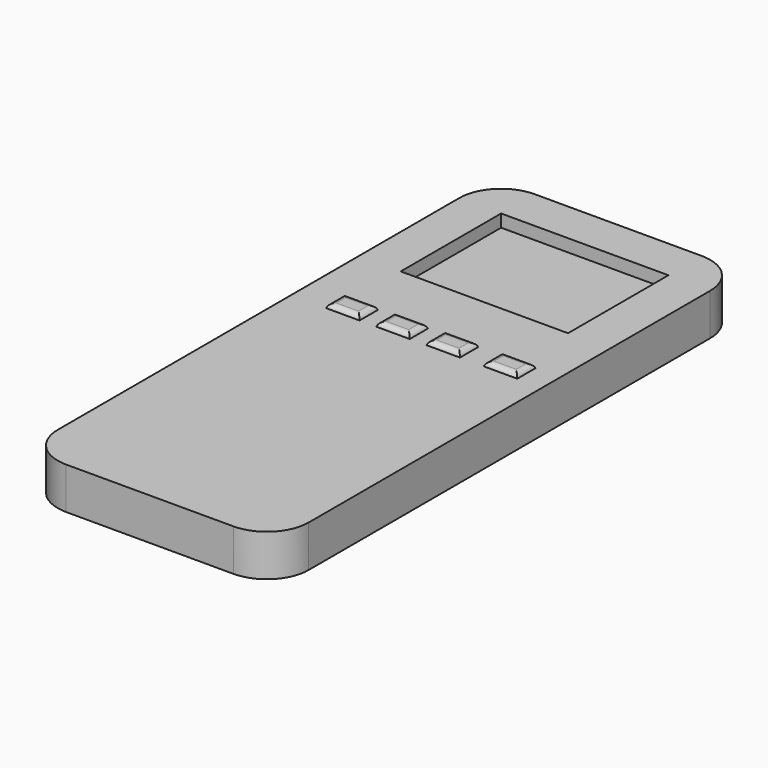
from build123d import *

# Parameters (mm, degrees)
F0_W        = 50.8
F0_H        = 38.1
F1_DEPTH    = 12.7
F2_DEPTH    = 8.89
F3_W        = 10.16
F3_H        = 6.9189891219
F3_H_2      = 6.9088
F4_DEPTH    = 1.27
F5_T1_DEPTH = 18.6794189943
F5_T3_DEPTH = 15.4384081162
F6_T1_DEPTH = 15.4384081162
F6_T3_DEPTH = 18.6794189943
F6_T5_DEPTH = 18.6794189943
F6_T7_DEPTH = 18.6794189943
F6_T9_DEPTH = 15.4282189943


# Not quite as in the source:
# - a fillet or chamfer that OpenCascade refuses, or shapes differently, is made with other operations: its cross-section is extruded or revolved along the edge and cut away or added


with BuildPart() as f1:
    # F0 (on Top) → F1 (new body)
    with BuildSketch(Plane.XY):
        with BuildLine():
            Line((26.8096346408, 46.6933250427), (-49.3903653592, 46.6933250427))
            Line((-49.3903653592, 46.6933250427), (-49.3903653592, -52.5104318142))
            ThreePointArc((-49.3903653592, -52.5104318142), (-45.6706214803, -61.4906879353), (-36.6903653592, -65.2104318142))
            Line((-36.6903653592, -65.2104318142), (14.1096346408, -65.2104318142))
            ThreePointArc((14.1096346408, -65.2104318142), (23.0898907619, -61.4906879353), (26.8096346408, -52.5104318142))
            Line((26.8096346408, -52.5104318142), (26.8096346408, 46.6933250427))
        make_face()
        with BuildLine():
            Line((14.1096346408, 112.5895681858), (-36.6903653592, 112.5895681858))
            ThreePointArc((-36.6903653592, 112.5895681858), (-45.6706214803, 108.8698243069), (-49.3903653592, 99.8895681858))
            Line((-49.3903653592, 99.8895681858), (-49.3903653592, 46.6933250427))
            Line((-49.3903653592, 46.6933250427), (26.8096346408, 46.6933250427))
            Line((26.8096346408, 46.6933250427), (26.8096346408, 99.8895681858))
            ThreePointArc((26.8096346408, 99.8895681858), (23.0898907619, 108.8698243069), (14.1096346408, 112.5895681858))
        make_face()
        with Locations((-11.2903653592, 80.8395681858)):
            Rectangle(F0_W, F0_H, mode=Mode.SUBTRACT)
    extrude(amount=F1_DEPTH)

    # F0 (on Top) → F2 (join)
    with BuildSketch(Plane.XY):
        with Locations((-11.2903653592, 80.8395681858)):
            Rectangle(F0_W, F0_H)
    extrude(amount=F2_DEPTH)

    # F3 (on face) → F4 (join)
    with BuildSketch(Plane.XY.offset(12.7)):
        with Locations((-33.6411841828, 39.4687093794)):
            Rectangle(F3_W, F3_H)
        with Locations((-18.4011841828, 39.4687093794)):
            Rectangle(F3_W, F3_H)
        with Locations((-3.1611841828, 39.4738039404)):
            Rectangle(F3_W, F3_H_2)
        with Locations((14.2273069042, 39.4738039404)):
            Rectangle(F3_W, F3_H_2)
    extrude(amount=F4_DEPTH)

    # F5: fillet of radius 1.778 on 4 edges, made by hand

    # F5_s2 → F5_t1 (cut)
    with BuildSketch(Plane.YZ.offset(-42.9808936799)):
        with BuildLine():
            ThreePointArc((42.9282039404, 12.7), (42.2868783752, 13.6175714644), (41.2243201415, 13.97))
            Line((41.2243201415, 13.97), (42.9282039404, 13.97))
            Line((42.9282039404, 13.97), (42.9282039404, 12.7))
        make_face()
        with BuildLine():
            ThreePointArc((36.0092148185, 12.7), (36.6505403836, 13.6175714644), (37.7130986173, 13.97))
            Line((37.7130986173, 13.97), (36.0092148185, 13.97))
            Line((36.0092148185, 13.97), (36.0092148185, 12.7))
        make_face()
    extrude(amount=F5_T1_DEPTH, mode=Mode.SUBTRACT)

    # F5_s4 → F5_t3 (cut)
    with BuildSketch(Plane.XZ.offset(-47.1879134375)):
        with BuildLine():
            ThreePointArc((-38.7211841828, 12.7), (-38.0798586176, 13.6175714644), (-37.0173003839, 13.97))
            Line((-37.0173003839, 13.97), (-38.7211841828, 13.97))
            Line((-38.7211841828, 13.97), (-38.7211841828, 12.7))
        make_face()
        with BuildLine():
            ThreePointArc((-28.5611841828, 12.7), (-29.2025097479, 13.6175714644), (-30.2650679816, 13.97))
            Line((-30.2650679816, 13.97), (-28.5611841828, 13.97))
            Line((-28.5611841828, 13.97), (-28.5611841828, 12.7))
        make_face()
    extrude(amount=F5_T3_DEPTH, mode=Mode.SUBTRACT)

    # F6: fillet of radius 1.778 on 12 edges, made by hand

    # F6_s2 → F6_t1 (cut)
    with BuildSketch(Plane.XZ.offset(-47.1879134375)):
        with BuildLine():
            ThreePointArc((-23.4811841828, 12.7), (-22.8398586176, 13.6175714644), (-21.7773003839, 13.97))
            Line((-21.7773003839, 13.97), (-23.4811841828, 13.97))
            Line((-23.4811841828, 13.97), (-23.4811841828, 12.7))
        make_face()
        with BuildLine():
            ThreePointArc((-13.3211841828, 12.7), (-13.9625097479, 13.6175714644), (-15.0250679816, 13.97))
            Line((-15.0250679816, 13.97), (-13.3211841828, 13.97))
            Line((-13.3211841828, 13.97), (-13.3211841828, 12.7))
        make_face()
    extrude(amount=F6_T1_DEPTH, mode=Mode.SUBTRACT)

    # F6_s4 → F6_t3 (cut)
    with BuildSketch(Plane.YZ.offset(-27.7408936799)):
        with BuildLine():
            ThreePointArc((36.0092148185, 12.7), (36.6505403836, 13.6175714644), (37.7130986173, 13.97))
            Line((37.7130986173, 13.97), (36.0092148185, 13.97))
            Line((36.0092148185, 13.97), (36.0092148185, 12.7))
        make_face()
        with BuildLine():
            ThreePointArc((42.9282039404, 12.7), (42.2868783752, 13.6175714644), (41.2243201415, 13.97))
            Line((41.2243201415, 13.97), (42.9282039404, 13.97))
            Line((42.9282039404, 13.97), (42.9282039404, 12.7))
        make_face()
    extrude(amount=F6_T3_DEPTH, mode=Mode.SUBTRACT)

    # F6_s6 → F6_t5 (cut)
    with BuildSketch(Plane.YZ.offset(-12.5008936799)):
        with BuildLine():
            ThreePointArc((42.9282039404, 12.7), (42.2868783752, 13.6175714644), (41.2243201415, 13.97))
            Line((41.2243201415, 13.97), (42.9282039404, 13.97))
            Line((42.9282039404, 13.97), (42.9282039404, 12.7))
        make_face()
        with BuildLine():
            ThreePointArc((36.0194039404, 12.7), (36.6607295055, 13.6175714644), (37.7232877392, 13.97))
            Line((37.7232877392, 13.97), (36.0194039404, 13.97))
            Line((36.0194039404, 13.97), (36.0194039404, 12.7))
        make_face()
    extrude(amount=F6_T5_DEPTH, mode=Mode.SUBTRACT)

    # F6_s8 → F6_t7 (cut)
    with BuildSketch(Plane.YZ.offset(4.8875974071)):
        with BuildLine():
            ThreePointArc((42.9282039404, 12.7), (42.2868783752, 13.6175714644), (41.2243201415, 13.97))
            Line((41.2243201415, 13.97), (42.9282039404, 13.97))
            Line((42.9282039404, 13.97), (42.9282039404, 12.7))
        make_face()
        with BuildLine():
            ThreePointArc((36.0194039404, 12.7), (36.6607295055, 13.6175714644), (37.7232877392, 13.97))
            Line((37.7232877392, 13.97), (36.0194039404, 13.97))
            Line((36.0194039404, 13.97), (36.0194039404, 12.7))
        make_face()
    extrude(amount=F6_T7_DEPTH, mode=Mode.SUBTRACT)

    # F6_s10 → F6_t9 (cut)
    with BuildSketch(Plane.XZ.offset(-47.1879134375)):
        with BuildLine():
            ThreePointArc((9.1473069042, 12.7), (9.7886324694, 13.6175714644), (10.8511907031, 13.97))
            Line((10.8511907031, 13.97), (9.1473069042, 13.97))
            Line((9.1473069042, 13.97), (9.1473069042, 12.7))
        make_face()
        with BuildLine():
            ThreePointArc((19.3073069042, 12.7), (18.665981339, 13.6175714644), (17.6034231053, 13.97))
            Line((17.6034231053, 13.97), (19.3073069042, 13.97))
            Line((19.3073069042, 13.97), (19.3073069042, 12.7))
        make_face()
        with BuildLine():
            ThreePointArc((-8.2411841828, 12.7), (-7.5998586176, 13.6175714644), (-6.5373003839, 13.97))
            Line((-6.5373003839, 13.97), (-8.2411841828, 13.97))
            Line((-8.2411841828, 13.97), (-8.2411841828, 12.7))
        make_face()
        with BuildLine():
            ThreePointArc((1.9188158172, 12.7), (1.2774902521, 13.6175714644), (0.2149320184, 13.97))
            Line((0.2149320184, 13.97), (1.9188158172, 13.97))
            Line((1.9188158172, 13.97), (1.9188158172, 12.7))
        make_face()
    extrude(amount=F6_T9_DEPTH, mode=Mode.SUBTRACT)


solid = f1.part
